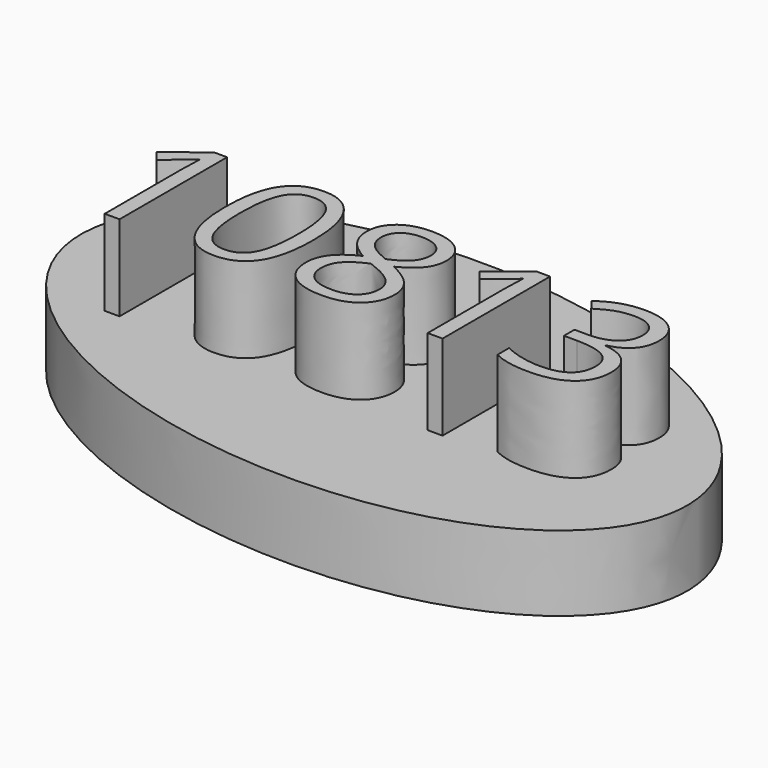
from build123d import *

# Parameters (mm, degrees)
F1_DEPTH     = 28.194
F2_TEXT_SIZE = 70.4985448263
F3_DEPTH     = 32.004


# Not quite as in the source:
# - Text() gives the source's letters only with a copy of the font that has no kerning and outlines rounded to 1/6400 em; it was checked with that copy


with BuildPart() as f1:
    # F0 (on Top) → F1 (new body)
    with BuildSketch(Plane.XY):
        with BuildLine():
            add(Edge.make_bspline(
                [(-122.4717721343, 17.0614942908), (-139.0598863846, -102.0122347724), (52.941828942, -68.067611677), (244.9435442686, -34.1229885817), (69.5299431923, 51.0061173862), (-105.883657884, 136.1352233541), (-122.4717721343, 17.0614942908)],
                knots=[0, 0, 0, 2.0943951024, 2.0943951024, 4.1887902048, 4.1887902048, 6.2831853072, 6.2831853072, 6.2831853072], degree=2, weights=[1, 0.5, 1, 0.5, 1, 0.5, 1]))
        make_face()
    extrude(amount=F1_DEPTH)

    # F2 (on face) → F3 (join)
    with BuildSketch(Plane.XY.offset(28.194)):
        with Locations((-106.139505282, -21.8302290887)):
            Text('10813', F2_TEXT_SIZE, font='Open Sans', text_align=(TextAlign.LEFT, TextAlign.BOTTOM))
    extrude(amount=F3_DEPTH)


solid = f1.part
